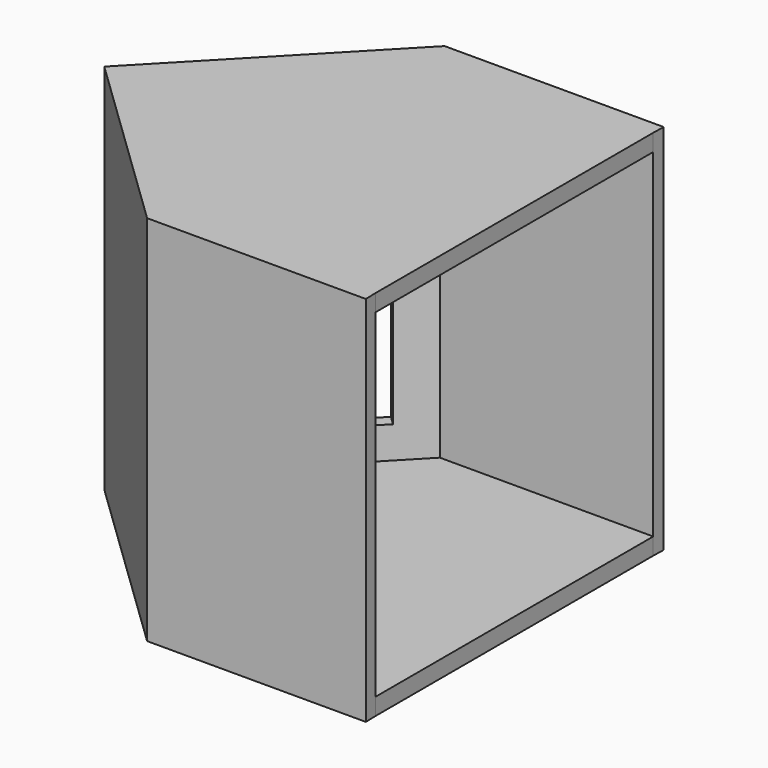
from build123d import *

# Parameters (mm, degrees)
F1_DEPTH  = 40
F2_DEPTH  = 2
F3_DEPTH  = 2
F4_W      = 25.2149685806
F4_H      = 2
F5_DEPTH  = 42.1
F5_FACE_W = 40.9870653462
F5_FACE_H = 2
F7_W      = 25.2149685806
F7_H      = 2
F8_DEPTH  = 42
F8_FACE_W = 40.9870653462
F8_FACE_H = 2
F10_W     = 21.6691600519
F10_H     = 33.2297814414
F11_DEPTH = 5.3


with BuildPart() as f1:
    # F0 (on Top) → F1 (new body)
    with BuildSketch(Plane.XY):
        Polygon((-13.4906232357, 20.567771814), (-24.4906232357, 20.567771814), (-39.384083382, 20.567771814), (-61.3453843386, -2.2496986568), (-39.33704599, -23.432228186), (-13.4906232357, -23.432228186), (-13.530928939, -21.9322283479), (-38.732458267, -21.9322283479), (-59.2244518674, -2.2091464562), (-38.7458975196, 19.0677719759), (-24.530928939, 19.0677719759), (-13.530928939, 19.0677719759), align=None)
    extrude(amount=F1_DEPTH)

    # F2 (add): a face of the model
    f2_faces = [f1.faces().sort_by_distance(p)[0] for p in [
        (-49.4292616832, -12.5390688822, 40),
    ]]
    extrude(f2_faces, amount=F2_DEPTH)

    # F3 (add): a face of the model
    f3_faces = [f1.faces().sort_by_distance(p)[0] for p in [
        (-49.4292616832, -12.5390688822, 42),
    ]]
    extrude(f3_faces, amount=F3_DEPTH)

    # F4 (on face) → F5 (join)
    with BuildSketch(Plane.XZ.offset(-19.0677719759)):
        with Locations((-26.1384132293, 43)):
            Rectangle(F4_W, F4_H)
    extrude(amount=F5_DEPTH)

    # F5_face (on face) → F6 (join, up to the next surface of F1)
    with BuildSketch(Plane(origin=(-38.7458975196, -1.4257606972, 43), x_dir=(0, -1, 0), z_dir=(-1, 0, 0))):
        Rectangle(F5_FACE_W, F5_FACE_H)
    extrude(until=Until.NEXT)

    # F7 (on face) → F8 (join)
    with BuildSketch(Plane.XZ.offset(-19.0677719759)):
        with Locations((-26.1384132293, 1)):
            Rectangle(F7_W, F7_H)
    extrude(amount=F8_DEPTH)

    # F8_face (on face) → F9 (join, up to the next surface of F1)
    with BuildSketch(Plane(origin=(-38.7458975196, -1.4257606972, 1), x_dir=(0, -1, 0), z_dir=(-1, 0, 0))):
        Rectangle(F8_FACE_W, F8_FACE_H)
    extrude(until=Until.NEXT)

    # F10 (on face) → F11 (cut)
    with BuildSketch(Plane(origin=(-30.7211592709, 29.5684232548, 0), x_dir=(-0.6934601651, -0.7204949684, 0), z_dir=(-0.7204949684, 0.6934601651, 0))):
        with Locations((28.3268968852, 22.3851092793)):
            Rectangle(F10_W, F10_H)
    extrude(amount=-F11_DEPTH, mode=Mode.SUBTRACT)


solid = f1.part
